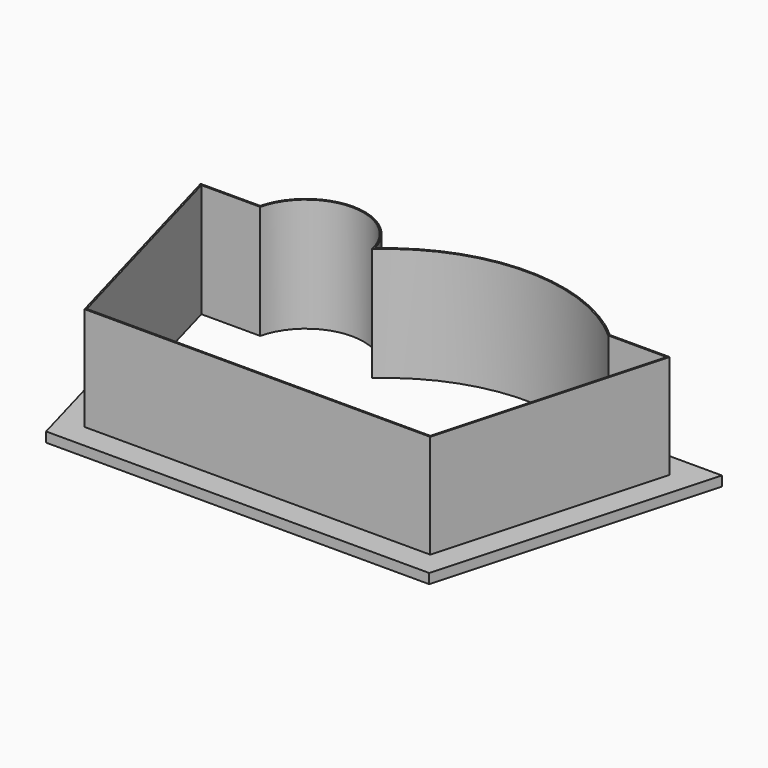
from build123d import *

# Parameters (mm, degrees)
F2_DEPTH = 2
F3_DEPTH = 23
F5_DEPTH = 23


# Not quite as in the source:
# - a feature of the source that left no trace in its solid (it failed there, or was rolled back) is left out


with BuildPart() as f2:
    # F1 (on Top) → F2 (new body)
    with BuildSketch(Plane.XY):
        with BuildLine():
            ThreePointArc((37.2509612746, 50), (13.7972702688, 58.9420922887), (-10.4728523554, 52.5391410864))
            ThreePointArc((-10.4728523554, 52.5391410864), (-25.3288691863, 58.932170126), (-38.8117617996, 50))
            Line((-38.8117617996, 50), (-54.0782060256, 50))
            Line((-54.0782060256, 50), (-38.8004282479, -5))
            Line((-38.8004282479, -5), (38.8004282479, -5))
            Line((38.8004282479, -5), (54.0782060256, 50))
            Line((54.0782060256, 50), (37.2509612746, 50))
        make_face()
    extrude(amount=F2_DEPTH)

    # F0 (on Top) → F3 (join)
    with BuildSketch(Plane.XY):
        with BuildLine():
            Line((-35.4307118382, 45), (-47.5, 45))
            Line((-47.5, 45), (-35, 0))
            Line((-35, 0), (35, 0))
            Line((35, 0), (47.5, 45))
            Line((47.5, 45), (35.4307118382, 45))
            ThreePointArc((35.4307118382, 45), (11.6189500386, 54), (-12.192811761, 45))
            ThreePointArc((-12.192811761, 45), (-23.8117617996, 54), (-35.4307118382, 45))
        make_face()
    extrude(amount=F3_DEPTH)

    # F4 (on face) → F5 (cut, through all)
    with BuildSketch(Plane.XY.offset(23)):
        with BuildLine():
            ThreePointArc((35.3170512284, 44.7), (11.4242314878, 53.6994689692), (-12.3689964911, 44.4399020665))
            ThreePointArc((-12.3689964911, 44.4399020665), (-23.678456811, 53.6992405642), (-35.1959613762, 44.7))
            Line((-35.1959613762, 44.7), (-47.1053076385, 44.7))
            Line((-47.1053076385, 44.7), (-34.7719743051, 0.3))
            Line((-34.7719743051, 0.3), (34.7719743051, 0.3))
            Line((34.7719743051, 0.3), (47.1053076385, 44.7))
            Line((47.1053076385, 44.7), (35.3170512284, 44.7))
        make_face()
    extrude(amount=-F5_DEPTH, mode=Mode.SUBTRACT)


solid = f2.part
